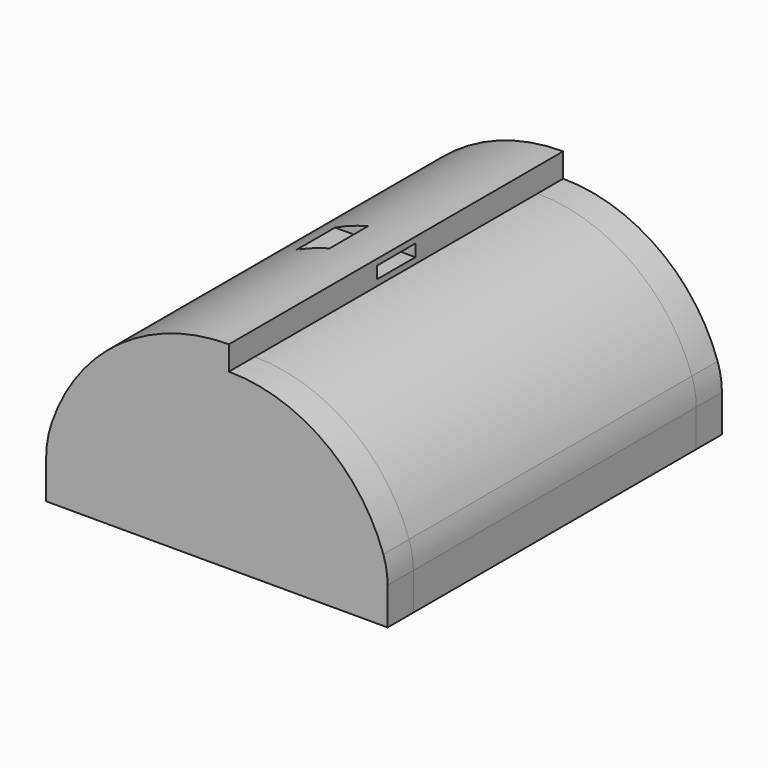
from build123d import *

# Parameters (mm, degrees)
F1_DEPTH = 22
F10_R    = 1
F11_R    = 10
F3_DEPTH = 4
F7_DEPTH = 52
F8_W     = 6
F8_H     = 1.5
F9_DEPTH = 25


# Not quite as in the source:
# - a feature of the source that left no trace in its solid (it failed there, or was rolled back) is left out


with BuildPart() as f1:
    # F0 (on Front) → F1 (new body, symmetric)
    with BuildSketch(Plane.XZ):
        with BuildLine():
            Line((13.45, 0), (7.75, 0))
            Line((7.75, 0), (7.75, -6))
            Line((7.75, -6), (19.75, -6))
            Line((19.75, -6), (19.75, 0))
            ThreePointArc((19.75, 0), (12.583943142, 11.2295914778), (0, 15.6))
            Line((0, 15.6), (0, 9.6))
            ThreePointArc((0, 9.6), (8.2623014348, 6.9538233644), (13.45, 0))
        make_face()
        with BuildLine():
            ThreePointArc((-13.45, 0), (-8.2623014348, 6.9538233644), (0, 9.6))
            Line((0, 9.6), (0, 15.6))
            ThreePointArc((0, 15.6), (-12.583943142, 11.2295914778), (-19.75, 0))
            Line((-19.75, 0), (-19.75, -6))
            Line((-19.75, -6), (-7.75, -6))
            Line((-7.75, -6), (-7.75, 0))
            Line((-7.75, 0), (-13.45, 0))
        make_face()
    extrude(amount=F1_DEPTH, both=True)

    # F10
    f10_edges = [f1.edges().sort_by_distance(p)[0] for p in [
        (-7.75, 0, -6),
        (-7.75, 0, 0),
        (7.75, 0, 0),
        (7.75, 0, -6),
    ]]
    fillet(f10_edges, radius=F10_R)

    # F11
    f11_edges = [f1.edges().sort_by_distance(p)[0] for p in [
        (19.75, 0, 0),
        (-19.75, 0, 0),
    ]]
    fillet(f11_edges, radius=F11_R)


with BuildPart() as f3:
    # F2 (on face) → F3 (new body)
    with BuildSketch(Plane.XZ.offset(22)):
        with BuildLine():
            ThreePointArc((19.75, -1.3750270948), (19.6151352671, 0.2617704372), (19.2141787678, 1.8544187169))
            ThreePointArc((19.2141787678, 1.8544187169), (0, 15.6), (-19.2141787678, 1.8544187169))
            ThreePointArc((-19.2141787678, 1.8544187169), (-19.6151352671, 0.2617704372), (-19.75, -1.3750270948))
            Line((-19.75, -1.3750270948), (-19.75, -6))
            Line((-19.75, -6), (-8.75, -6))
            Line((-8.75, -6), (8.75, -6))
            Line((8.75, -6), (19.75, -6))
            Line((19.75, -6), (19.75, -1.3750270948))
        make_face()
    extrude(amount=F3_DEPTH)


with BuildPart() as f12_1:
    # F12: instance of F3
    add(f3.part.mirror(Plane.XZ))


with BuildPart() as f3_1:
    add(f3.part)

    add(f12_1.part)  # F7 merges F12_1
    # F6 (on face) → F7 (join, through all)
    with BuildSketch(Plane.XZ.offset(26)):
        with BuildLine():
            ThreePointArc((0, 18.6), (-13.5578357737, 14.2497366228), (-22.0534323982, 2.8232524604))
            ThreePointArc((-22.0534323982, 2.8232524604), (-22.5746758473, 0.7528096968), (-22.75, -1.3750270948))
            Line((-22.75, -1.3750270948), (-22.75, -6))
            Line((-22.75, -6), (-19.75, -6))
            Line((-19.75, -6), (-19.75, -1.3750270948))
            ThreePointArc((-19.75, -1.3750270948), (-19.6151352671, 0.2617704372), (-19.2141787678, 1.8544187169))
            ThreePointArc((-19.2141787678, 1.8544187169), (-11.8123417506, 11.8098082191), (0, 15.6))
            Line((0, 15.6), (0, 18.6))
        make_face()
    extrude(amount=-F7_DEPTH)

    # F8 (on face) → F9 (cut)
    with BuildSketch(Plane.YZ):
        with Locations((0, 17.0999999998)):
            Rectangle(F8_W, F8_H)
    extrude(amount=-F9_DEPTH, mode=Mode.SUBTRACT)


solid = Compound([f1.part, f3_1.part])
